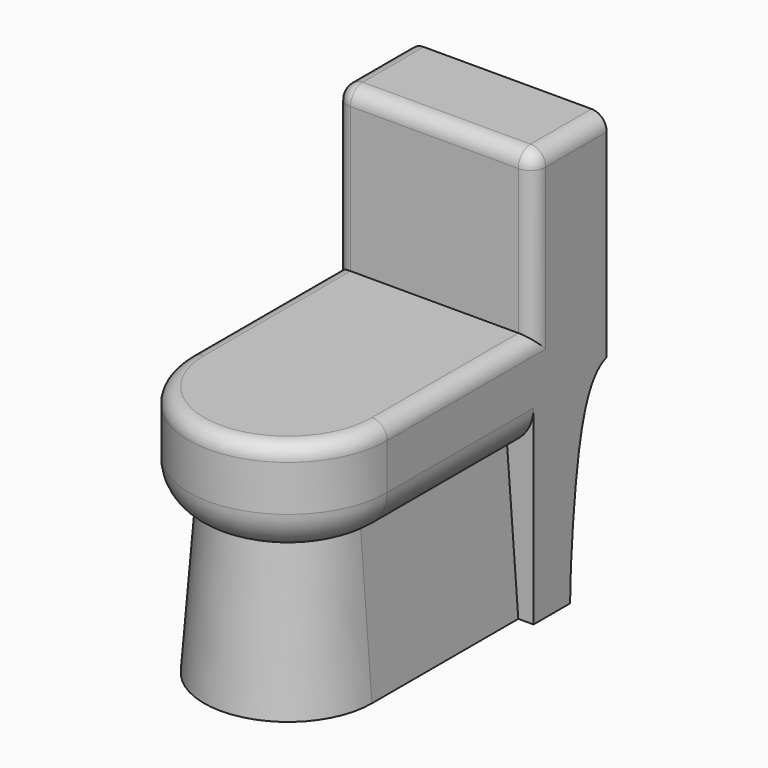
from build123d import *

# Parameters (mm, degrees)
F0_R          = 12.7
F1_DEPTH      = 419.1
F0_W          = 165.1
F0_H          = 152.4
F2_DEPTH      = 685.8
F3_DEPTH      = 25.4
F8_DEPTH      = 165.1010001
F8_DEPTH_BACK = 165.1010001
F9_R          = 25.4


with BuildPart() as f1:
    # F0 (on Top) → F1 (new body)
    with BuildSketch(Plane.XY):
        with BuildLine():
            Line((0, -266.7), (0, -152.4))
            Line((0, -152.4), (-165.1, -152.4))
            Line((-165.1, -152.4), (-165.1, -457.2))
            ThreePointArc((-165.1, -457.2), (-116.7433295739, -573.9433295739), (0, -622.3))
            Line((0, -622.3), (0, -342.9))
            ThreePointArc((0, -342.9), (-38.1, -304.8), (0, -266.7))
        make_face()
        with Locations((-101.6, -203.2)):
            Circle(F0_R, mode=Mode.SUBTRACT)
        with Locations((-101.6, -203.2)):
            Circle(F0_R)
        with BuildLine():
            Line((0, -342.9), (0, -266.7))
            ThreePointArc((0, -266.7), (-38.1, -304.8), (0, -342.9))
        make_face()
    extrude(amount=F1_DEPTH)

    # F0 (on Top) → F2 (join)
    with BuildSketch(Plane.XY):
        with Locations((-82.55, -76.2)):
            Rectangle(F0_W, F0_H)
    extrude(amount=F2_DEPTH)

    # F0 (on Top) → F3 (cut)
    with BuildSketch(Plane.XY):
        with BuildLine():
            Line((0, -342.9), (0, -266.7))
            ThreePointArc((0, -266.7), (-38.1, -304.8), (0, -342.9))
        make_face()
    extrude(amount=F3_DEPTH, mode=Mode.SUBTRACT)

    # F4: F1 across face


with BuildPart() as f1_1:
    add(f1.part)
    add(f1.part.mirror(Plane(origin=(0, -279.3076736672, 257.3545234249), x_dir=(0, 1, 0), z_dir=(1, 0, 0))))

    # F6: sweep along a path in F6_path
    with BuildLine(Plane(origin=(-165.1, -152.4, 419.1), x_dir=(0, 1, 0), z_dir=(0, 0, 1))) as f6_path:
        Line((0, 0), (-304.8, 0))
        ThreePointArc((-304.8, 0), (-469.9, -165.1), (-304.8, -330.2))
        Line((-304.8, -330.2), (0, -330.2))
    # F5 (on face) → F6 (sweep, cut)
    with BuildSketch(Plane.XZ.offset(152.4)):
        with BuildLine():
            ThreePointArc((-120.65, 254), (-152.8833058285, 278.74418592), (-165.1, 317.5))
            Line((-165.1, 317.5), (-165.1, 0))
            Line((-165.1, 0), (-139.7, 0))
            Line((-139.7, 0), (-120.65, 254))
        make_face()
    sweep(path=f6_path.line, mode=Mode.SUBTRACT)

    # F7 (on Right) → F8 (cut, two sides)
    with BuildSketch(Plane.YZ) as f8_sk:
        with BuildLine():
            add(Edge.make_bspline(
                [(-76.2, 0), (-76.2, 31.8793983715), (-69.0790448855, 184.3952112859), (-38.761105776, 317.4984685435), (0, 330.2)],
                knots=[0, 0, 0, 0, 0.5205513628, 1, 1, 1, 1], degree=3))
            Line((-76.2, 0), (0, 0))
            Line((0, 0), (0, 330.2))
        make_face()
    extrude(amount=-F8_DEPTH, mode=Mode.SUBTRACT)
    extrude(f8_sk.sketch, amount=F8_DEPTH_BACK, mode=Mode.SUBTRACT)

    # F9
    f9_edges = [f1_1.edges().sort_by_distance(p)[0] for p in [
        (-165.1, -76.2, 685.8),
        (-165.1, -152.4, 552.45),
        (0, -152.4, 685.8),
        (165.1, -76.2, 685.8),
        (165.1, -152.4, 552.45),
        (165.1, -304.8, 419.1),
        (0, -622.3, 419.1),
        (-165.1, -304.8, 419.1),
    ]]
    fillet(f9_edges, radius=F9_R)


solid = f1_1.part
